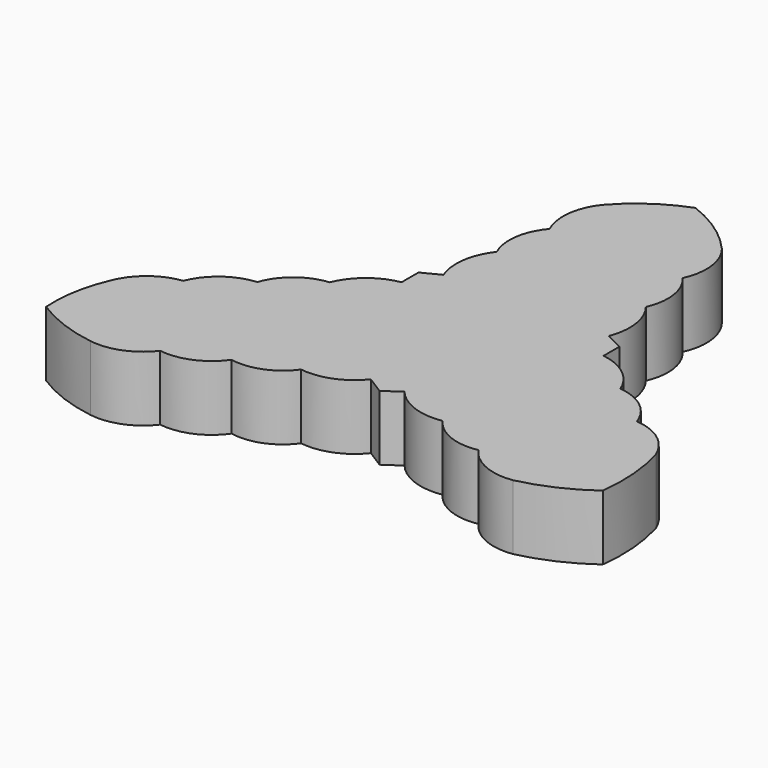
from build123d import *

# Parameters (mm, degrees)
F1_DEPTH = 7.9375


# Not quite as in the source:
# - a length typed as a fraction of an inch, garbled in the dataset ("3 / 203.2 mm" for 3/8 in), is restored


with BuildPart() as f1:
    # F0 (on Top) → F1 (new body)
    with BuildSketch(Plane.XY):
        with BuildLine():
            ThreePointArc((-0.0986067535, 34.0497419238), (-4.0682176485, 31.9659465467), (-7.4162920937, 28.9842672646))
            ThreePointArc((-7.4162920937, 28.9842672646), (-8.8119305122, 25.5953281623), (-8.2258973271, 21.977417171))
            ThreePointArc((-8.2258973271, 21.977417171), (-9.7181261566, 18.698842434), (-9.2097157612, 15.1327075437))
            ThreePointArc((-9.2097157612, 15.1327075437), (-10.6205392688, 11.8246856933), (-10.2093555033, 8.2519613206))
            Line((-10.2093555033, 8.2519613206), (-12.369341217, 7.1464567445))
            Line((-12.369341217, 7.1464567445), (-12.369341217, 4.6386048198))
            Line((-12.369341217, 4.6386048198), (-12.369341217, 4.5682978211))
            ThreePointArc((-12.369341217, 4.5682978211), (-15.5930977879, 3.1185654947), (-17.7027139134, 0.2823972963))
            ThreePointArc((-17.7027139134, 0.2823972963), (-21.0452825194, -1.0603738309), (-23.1384971151, -3.9919692741))
            ThreePointArc((-23.1384971151, -3.9919692741), (-26.5647165348, -5.2934051439), (-28.80180468, -8.19653302))
            ThreePointArc((-28.80180468, -8.19653302), (-32.1117440701, -9.5846599904), (-34.254974256, -12.4637500588))
            ThreePointArc((-34.254974256, -12.4637500588), (-35.4454588739, -16.4293701566), (-35.6585793197, -20.564340055))
            ThreePointArc((-35.6585793197, -20.564340055), (-31.9389059128, -22.4150036937), (-27.9142765499, -23.4461606411))
            ThreePointArc((-27.9142765499, -23.4461606411), (-24.3492963179, -23.0296138883), (-21.4921734029, -20.8571857766))
            ThreePointArc((-21.4921734029, -20.8571857766), (-17.8594468391, -20.3713745504), (-15.0192606046, -18.054899429))
            ThreePointArc((-15.0192606046, -18.054899429), (-11.4338171794, -17.7079201351), (-8.5996589687, -15.484556372))
            ThreePointArc((-8.5996589687, -15.484556372), (-5.0294162563, -15.0523544446), (-2.1409380715, -12.9098966718))
            Line((-2.1409380715, -12.9098966718), (0, -14.2561570176))
            Line((0, -14.2561570176), (1.9696742658, -12.9098966718))
            ThreePointArc((1.9696742658, -12.9098966718), (4.9392756736, -15.0084468105), (8.560301624, -15.3410370587))
            ThreePointArc((8.560301624, -15.3410370587), (11.3944598347, -17.5644008218), (14.9799032599, -17.9113801157))
            ThreePointArc((14.9799032599, -17.9113801157), (17.8200894944, -20.2278552371), (21.4528160582, -20.7136664634))
            ThreePointArc((21.4528160582, -20.7136664634), (25.6558468929, -19.2922500665), (29.4813849032, -17.0447733253))
            ThreePointArc((29.4813849032, -17.0447733253), (29.5836204245, -12.511977875), (28.7624473353, -8.0530137067))
            ThreePointArc((28.7624473353, -8.0530137067), (26.5253591901, -5.1498858306), (23.0991397704, -3.8484499608))
            ThreePointArc((23.0991397704, -3.8484499608), (21.0059251747, -0.9168545176), (17.6633565687, 0.4259166096))
            ThreePointArc((17.6633565687, 0.4259166096), (15.4847616458, 3.3168082822), (12.1560195839, 4.739132713))
            Line((12.1560195839, 4.739132713), (12.1560195839, 7.1464567445))
            Line((12.1560195839, 7.1464567445), (9.9960338703, 8.2519613206))
            ThreePointArc((9.9960338703, 8.2519613206), (10.4072176357, 11.8246856933), (8.9963941282, 15.1327075437))
            ThreePointArc((8.9963941282, 15.1327075437), (9.5048045235, 18.698842434), (8.012575694, 21.977417171))
            ThreePointArc((8.012575694, 21.977417171), (8.5986088792, 25.5953281623), (7.2029704606, 28.9842672646))
            ThreePointArc((7.2029704606, 28.9842672646), (3.8655773676, 31.9687453881), (-0.0986067535, 34.0497419238))
        make_face()
    extrude(amount=F1_DEPTH)


solid = f1.part
